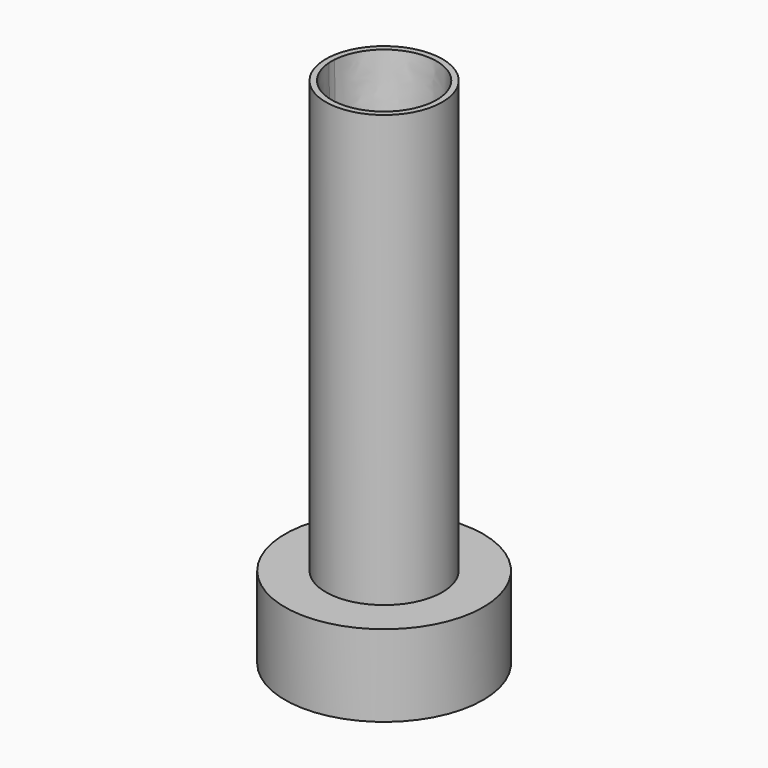
from build123d import *

# Parameters (mm, degrees)
F0_R         = 8.5
F1_DEPTH     = 7
F2_R         = 5
F6_DEPTH     = 37
F3_W         = 8
F3_H         = 0.2
F8_TEXT_SIZE = 4.7950337151
F9_DEPTH     = 0.2


# Not quite as in the source:
# - Text() gives the source's letters only with a copy of the font that has no kerning and outlines rounded to 1/6400 em; it was checked with that copy


with BuildPart() as f1:
    # F0 (on Top) → F1 (new body)
    with BuildSketch(Plane.XY):
        Circle(F0_R)
    extrude(amount=F1_DEPTH)

    # F2 (on face) → F6 (join)
    with BuildSketch(Plane.XY.offset(7)):
        Circle(F2_R)
    extrude(amount=F6_DEPTH)

    # F3 (on face) → F7 section 0
    with BuildSketch(Plane(origin=(0, 0, 0), x_dir=(1, 0, 0), z_dir=(0, 0, -1))):
        Rectangle(F3_W, F3_H)
    # F5 (on offset) → F7 section 1
    with BuildSketch(Plane.XY.offset(44)):
        with BuildLine():
            ThreePointArc((-4.4894398742, 0.3081065009), (-4.4999989228, 0.0031136609), (-4.4898619483, -0.3018934991))
            ThreePointArc((-4.4898619483, -0.3018934991), (0.003488119, -4.4999986481), (4.4903245708, -0.2949326172))
            ThreePointArc((4.4903245708, -0.2949326172), (4.4999886884, 0.0100898182), (4.4889568399, 0.3150658494))
            ThreePointArc((4.4889568399, 0.3150658494), (-0.0034880458, 4.4999986482), (-4.4894398742, 0.3081065009))
        make_face()
    loft(mode=Mode.SUBTRACT)

    # F8 (on face) → F9 (cut)
    with BuildSketch(Plane(origin=(0, 0, 0), x_dir=(1, 0, 0), z_dir=(0, 0, -1))):
        with Locations((-3.5, 1.5304341036)):
            Text('0.2', F8_TEXT_SIZE, font='Open Sans', font_style=FontStyle.BOLD, text_align=(TextAlign.LEFT, TextAlign.BOTTOM))
    extrude(amount=-F9_DEPTH, mode=Mode.SUBTRACT)


solid = f1.part
